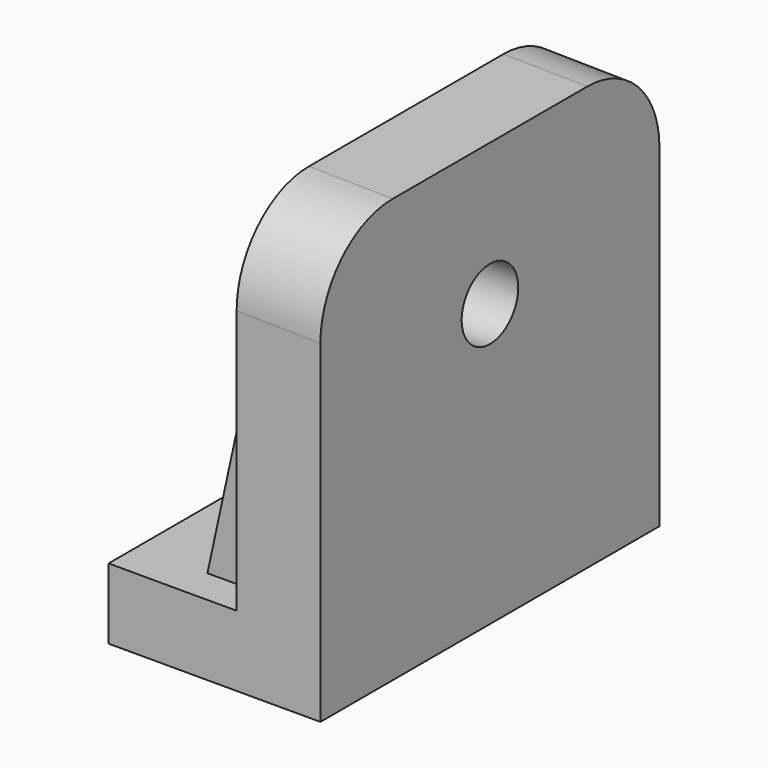
from build123d import *

# Parameters (mm, degrees)
F1_DEPTH       = 76.2
F3_DEPTH       = 25.4
F4_R           = 32.5001429767
F8_D           = 25.4
F8_CBORE_D     = 38.1
F8_CBORE_DEPTH = 6.35
F10_DEPTH      = 25.4
F12_DEPTH      = 25.4
F14_DEPTH      = 6.35


# Not quite as in the source:
# - a feature names something its author has since deleted; it is built from what else it names


with BuildPart() as f1:
    # F0 (on Front) → F1 (new body, symmetric)
    with BuildSketch(Plane.XZ):
        Polygon((5.1541254637, -56.7420329794), (5.1541254637, 95.6579670206), (-24.9778814614, 96.1331352592), (-24.9778814614, -31.3420329794), (-71.0458745363, -31.3420329794), (-71.0458745363, -56.7420329794), align=None)
    extrude(amount=F1_DEPTH, both=True)

    # F2 (on face) → F3 (cut)
    with BuildSketch(Plane.XY.offset(-31.3420329794)):
        with BuildLine():
            Line((-71.0458745363, 12.1218512269), (-71.0458745363, -13.2781487731))
            Line((-71.0458745363, -13.2781487731), (-58.3458745363, -13.2781487731))
            ThreePointArc((-58.3458745363, -13.2781487731), (-45.6458745363, -0.5781487731), (-58.3458745363, 12.1218512269))
            Line((-58.3458745363, 12.1218512269), (-71.0458745363, 12.1218512269))
        make_face()
    extrude(amount=-F3_DEPTH, mode=Mode.SUBTRACT)

    # F4
    f4_edges = [f1.edges().sort_by_distance(p)[0] for p in [
        (-9.911878, 76.2, 95.895551),
        (-9.911878, -76.2, 95.895551),
    ]]
    fillet(f4_edges, radius=F4_R)

    # F8 (through all)
    with Locations(Plane(origin=(-24.9778814614, 0, 0), x_dir=(0, -1, 0), z_dir=(-1, 0, 0))):
        with Locations((0, 44.6130335331)):
            CounterBoreHole(F8_D / 2, F8_CBORE_D / 2, F8_CBORE_DEPTH)

    # F9 (on face) → F10 (join)
    with BuildSketch(Plane.XZ.offset(38.1)):
        Polygon((-24.9547883868, -31.3420329794), (-24.9778814614, 63.6289514861), (-45.6458745363, -31.3420329794), align=None)
    extrude(amount=F10_DEPTH)

    # F11 (on face) → F12 (join)
    with BuildSketch(Plane(origin=(0, 38.1, 0), x_dir=(-1, 0, 0), z_dir=(0, 1, 0))):
        Polygon((45.6458745363, -31.3420329794), (24.9778814614, 63.6289514861), (24.9778814614, -31.3420329794), align=None)
    extrude(amount=F12_DEPTH)

    # F13 (on face) → F14 (join)
    with BuildSketch(Plane.XY.offset(-31.3420329794)):
        with BuildLine():
            Line((-71.0458745363, 18.4718512269), (-71.0458745363, 12.1218512269))
            Line((-71.0458745363, 12.1218512269), (-58.3458745363, 12.1218512269))
            ThreePointArc((-58.3458745363, 12.1218512269), (-45.6458745363, -0.5781487731), (-58.3458745363, -13.2781487731))
            Line((-58.3458745363, -13.2781487731), (-71.0458745363, -13.2781487731))
            Line((-71.0458745363, -13.2781487731), (-71.0458745363, -19.6281487731))
            Line((-71.0458745363, -19.6281487731), (-58.3458745363, -19.6281487731))
            ThreePointArc((-58.3458745363, -19.6281487731), (-39.2958745363, -0.5781487731), (-58.3458745363, 18.4718512269))
            Line((-58.3458745363, 18.4718512269), (-71.0458745363, 18.4718512269))
        make_face()
    extrude(amount=F14_DEPTH)


solid = f1.part
